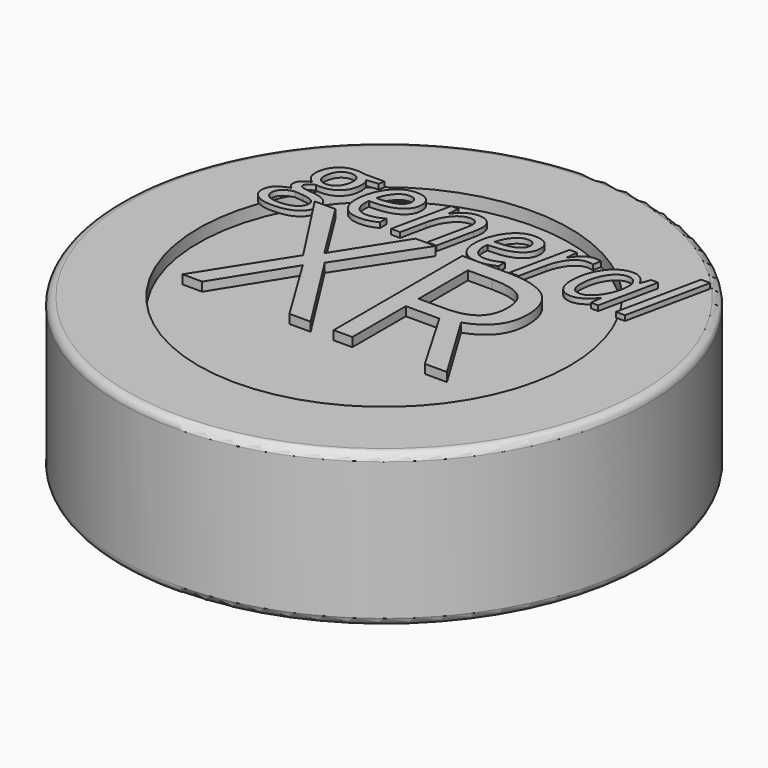
from build123d import *

# Parameters (mm, degrees)
F0_R         = 52.5427424817
F1_DEPTH     = 30.48
F2_R         = 1.524
F4_TEXT_SIZE = 44.8235297679
F5_DEPTH     = 1.778
F6_TEXT_SIZE = 22.0382353291
F7_DEPTH     = 1.016
F3_R         = 36.9698617404
F8_DEPTH     = 0.762
F9_DEPTH     = 1.778


# Not quite as in the source:
# - Text() gives the source's letters only with a copy of the font that has no kerning and outlines rounded to 1/6400 em; it was checked with that copy


with BuildPart() as f1:
    # F0 (on Top) → F1 (new body)
    with BuildSketch(Plane.XY):
        Circle(F0_R)
    extrude(amount=F1_DEPTH)

    # F2
    f2_edges = [f1.edges().sort_by_distance(p)[0] for p in [
        (-52.542742, 0, 30.48),
        (-52.542742, 0, 0),
    ]]
    fillet(f2_edges, radius=F2_R)

    # F4 (on face) → F5 (join)
    with BuildSketch(Plane.XY.offset(30.48)):
        with Locations((-27.2975303233, -16.2709411234)):
            Text('XR', F4_TEXT_SIZE, font='Open Sans', text_align=(TextAlign.LEFT, TextAlign.BOTTOM))
    extrude(amount=F5_DEPTH)

    # F6 (on face) → F7 (join)
    with BuildSketch(Plane.XY.offset(30.48)):
        with Locations((-34.8278842866, 17.0777644962)):
            Text('general', F6_TEXT_SIZE, font='Open Sans', font_style=FontStyle.ITALIC, text_align=(TextAlign.LEFT, TextAlign.BOTTOM))
    extrude(amount=F7_DEPTH)

    # F3 (on face) → F8 (cut)
    with BuildSketch(Plane.XY.offset(30.48)):
        Circle(F3_R)
    extrude(amount=-F8_DEPTH, mode=Mode.SUBTRACT)

    # F9 (cut): a face of the model
    f9_faces = [f1.faces().sort_by_distance(p)[0] for p in [
        (0, 0, 29.718),
    ]]
    extrude(f9_faces, amount=-F9_DEPTH, mode=Mode.SUBTRACT)


solid = f1.part
